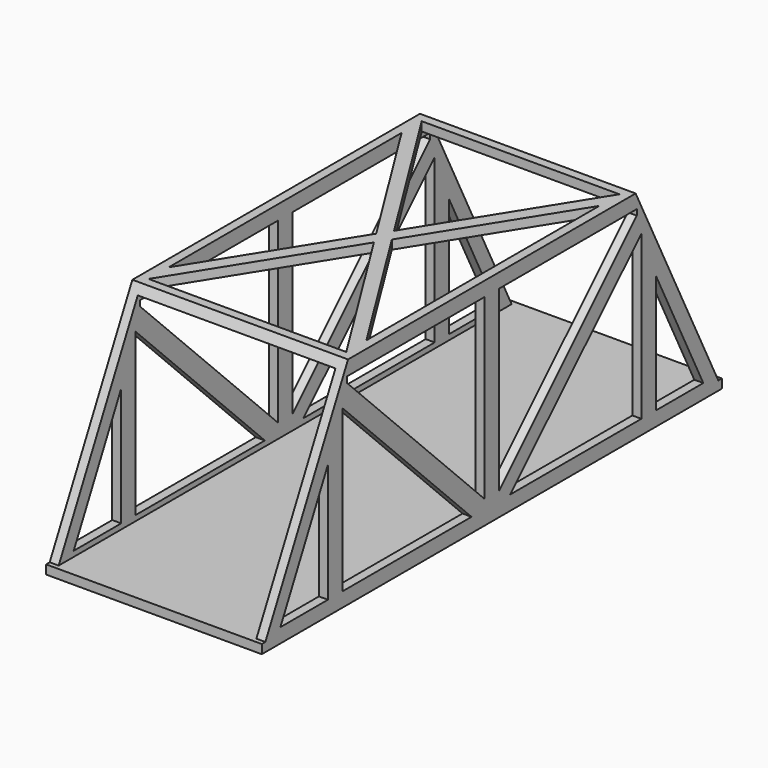
from build123d import *

# Parameters (mm, degrees)
F1_DEPTH = 38.1
F2_W     = 69.85
F2_H     = 69.85
F3_DEPTH = 127
F5_DEPTH = 76.2
F7_DEPTH = 5.588
F8_W     = 5.08
F8_H     = 3.175
F9_DEPTH = 76.2


with BuildPart() as f1:
    # F0 (on Right) → F1 (new body, symmetric)
    with BuildSketch(Plane.YZ):
        Polygon((-63.5, 32.0970378816), (-101.6, -44.1029621184), (101.6, -44.1029621184), (63.5, 32.0970378816), align=None)
    extrude(amount=F1_DEPTH, both=True)

    # F2 (on Front) → F3 (cut, symmetric)
    with BuildSketch(Plane.XZ):
        with Locations((0, -6.0029621184)):
            Rectangle(F2_W, F2_H)
    extrude(amount=F3_DEPTH, both=True, mode=Mode.SUBTRACT)

    # F4 (on face) → F5 (cut)
    with BuildSketch(Plane.YZ.offset(38.1)):
        Polygon((-72.39, 2.9578125559), (-93.3803873372, -39.0229621184), (-72.39, -39.0229621184), align=None)
        Polygon((-66.04, 18.0367817605), (-66.04, -39.0229621184), (-8.9802561211, -39.0229621184), align=None)
        Polygon((-3.175, 27.0170378816), (-64.008, 27.0170378816), (-64.008, 24.9850378816), (-3.175, -35.8479621184), align=None)
        Polygon((64.008, 27.0170378816), (3.175, 27.0170378816), (3.175, -35.8479621184), (64.008, 24.9850378816), align=None)
        Polygon((66.04, 18.5374412686), (8.0518, -39.0229621184), (66.04, -39.0229621184), align=None)
        Polygon((72.39, -39.0229621184), (93.3803873372, -39.0229621184), (72.39, 2.9578125559), align=None)
    extrude(amount=-F5_DEPTH, mode=Mode.SUBTRACT)

    # F6 (on face) → F7 (cut)
    with BuildSketch(Plane.XY.offset(32.0970378816)):
        Polygon((-34.925, 51.435), (-34.925, -51.435), (-2.778125, 0), align=None)
        Polygon((0, 4.445), (34.925, 60.325), (-34.925, 60.325), align=None)
        Polygon((2.778125, 0), (34.925, -51.435), (34.925, 51.435), align=None)
        Polygon((-34.925, -60.325), (34.925, -60.325), (0, -4.445), align=None)
    extrude(amount=-F7_DEPTH, mode=Mode.SUBTRACT)

    # F8 (on face) → F9 (join)
    with BuildSketch(Plane.YZ.offset(38.1)):
        with Locations((-99.06, -42.5154621184)):
            Rectangle(F8_W, F8_H)
        with Locations((99.06, -42.5154621184)):
            Rectangle(F8_W, F8_H)
    extrude(amount=-F9_DEPTH)


solid = f1.part
